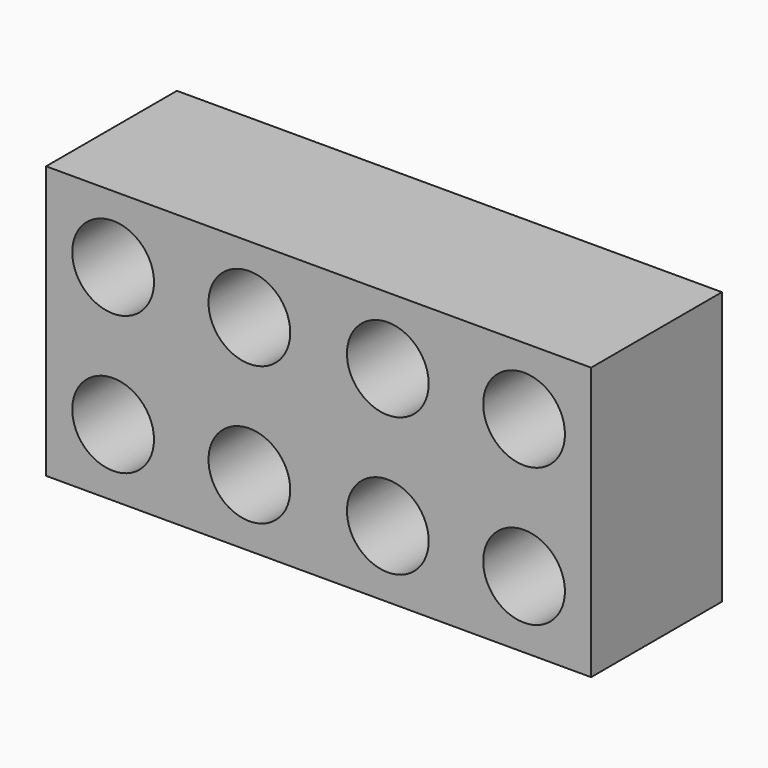
from build123d import *

# Parameters (mm, degrees)
F0_W     = 31.75
F0_H     = 15.875
F0_R     = 2.38125
F1_DEPTH = 9.525


# Not quite as in the source:
# - the program builds the solid bodies; features that only make, move or delete a surface that nothing else refers to are left out


with BuildPart() as f1:
    # F0 (on Front) → F1 (new body)
    with BuildSketch(Plane.XZ):
        with Locations((-15.875, -7.9375)):
            Rectangle(F0_W, F0_H)
        with Locations((-27.84475, -11.96975)):
            Circle(F0_R, mode=Mode.SUBTRACT)
        with Locations((-19.90725, -11.96975)):
            Circle(F0_R, mode=Mode.SUBTRACT)
        with Locations((-11.84275, -11.96975)):
            Circle(F0_R, mode=Mode.SUBTRACT)
        with Locations((-3.90525, -11.96975)):
            Circle(F0_R, mode=Mode.SUBTRACT)
        with Locations((-27.84475, -3.90525)):
            Circle(F0_R, mode=Mode.SUBTRACT)
        with Locations((-19.90725, -3.90525)):
            Circle(F0_R, mode=Mode.SUBTRACT)
        with Locations((-11.84275, -3.90525)):
            Circle(F0_R, mode=Mode.SUBTRACT)
        with Locations((-3.90525, -3.90525)):
            Circle(F0_R, mode=Mode.SUBTRACT)
    extrude(amount=F1_DEPTH)


solid = f1.part
